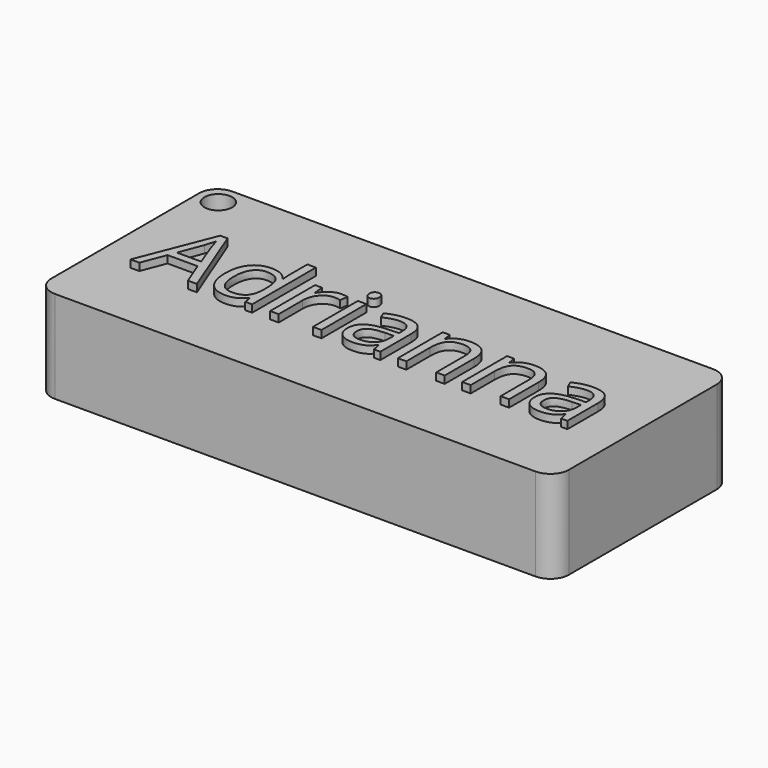
from build123d import *

# Parameters (mm, degrees)
F0_W         = 140
F0_H         = 60
F1_DEPTH     = 25
F2_TEXT_SIZE = 28.3656509695
F3_DEPTH     = 2
F4_R         = 3.75
F5_DEPTH     = 25
F6_R         = 5


# Not quite as in the source:
# - Text() gives the source's letters only with a copy of the font that has no kerning and outlines rounded to 1/6400 em; it was checked with that copy


with BuildPart() as f1:
    # F0 (on Top) → F1 (new body)
    with BuildSketch(Plane.XY):
        Rectangle(F0_W, F0_H)
    extrude(amount=F1_DEPTH)

    # F2 (on face) → F3 (join)
    with BuildSketch(Plane.XY.offset(25)):
        with Locations((-60, -10.7038579936)):
            Text('Adrianna', F2_TEXT_SIZE, font='Open Sans', text_align=(TextAlign.LEFT, TextAlign.BOTTOM))
    extrude(amount=F3_DEPTH)

    # F4 (on face) → F5 (cut)
    with BuildSketch(Plane.XY.offset(25)):
        with Locations((-64.2532259226, 24.3024174124)):
            Circle(F4_R)
    extrude(amount=-F5_DEPTH, mode=Mode.SUBTRACT)

    # F6
    f6_edges = [f1.edges().sort_by_distance(p)[0] for p in [
        (70, -30, 12.5),
        (-70, -30, 12.5),
        (70, 30, 12.5),
        (-70, 30, 12.5),
    ]]
    fillet(f6_edges, radius=F6_R)


solid = f1.part
